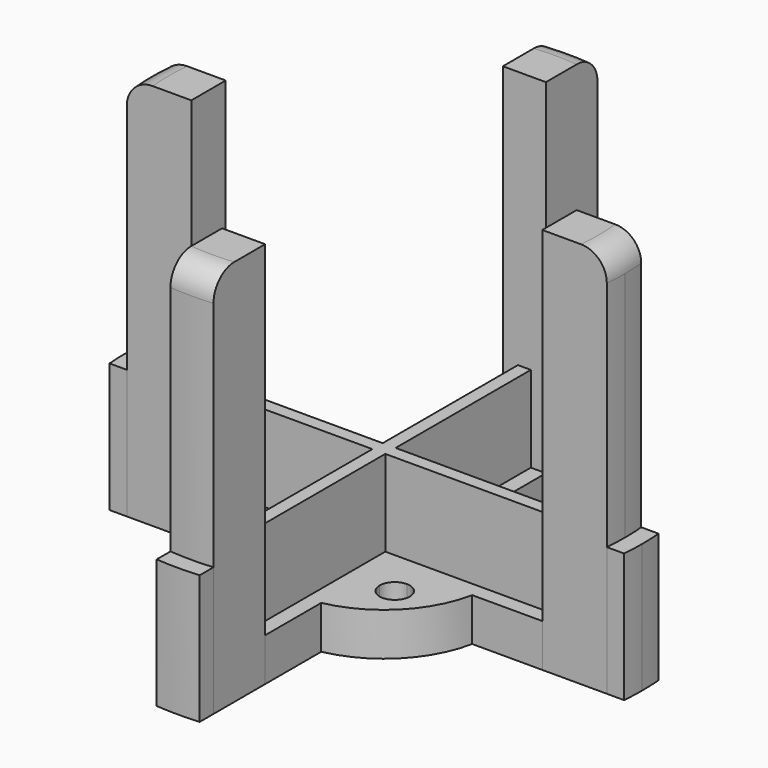
from build123d import *

# Parameters (mm, degrees)
F0_W          = 3.5
F0_H          = 7.5
F0_W_2        = 7.5
F0_H_2        = 3.5
F1_DEPTH      = 10
F0_W_3        = 3
F0_H_3        = 3
F2_DEPTH      = 30
F3_DEPTH      = 90
F4_T2_ANGLE   = 40.9393595263
F4_2_T2_ANGLE = 40.9393595263
F4_3_T2_ANGLE = 40.9393595263
F4_4_T2_ANGLE = 40.9393595263
F5_DEPTH      = 3


# Not quite as in the source:
# - a fillet or chamfer that OpenCascade refuses, or shapes differently, is made with other operations: its cross-section is extruded or revolved along the edge and cut away or added


with BuildPart() as f1:
    # F0 (on Top) → F1 (new body)
    with BuildSketch(Plane.XY):
        with BuildLine():
            Line((12.5, 5), (24.4948974278, 5))
            ThreePointArc((24.4948974278, 5), (17.6776695297, 17.6776695297), (5, 24.4948974278))
            Line((5, 24.4948974278), (5, 12.5))
            Line((5, 12.5), (9, 12.5))
            ThreePointArc((9, 12.5), (12.5, 16), (16, 12.5))
            ThreePointArc((16, 12.5), (14.9748737342, 10.0251262658), (12.5, 9))
            Line((12.5, 9), (12.5, 5))
        make_face()
        with BuildLine():
            Line((5, 12.5), (5, 24.4948974278))
            ThreePointArc((5, 24.4948974278), (3.2581304855, 24.7867824806), (1.5, 24.9549594269))
            Line((1.5, 24.9549594269), (1.5, 12.5))
            Line((1.5, 12.5), (5, 12.5))
        make_face()
        with Locations((3.25, 8.75)):
            Rectangle(F0_W, F0_H)
        with BuildLine():
            Line((5, 5), (12.5, 5))
            Line((12.5, 5), (12.5, 9))
            ThreePointArc((12.5, 9), (10.0251262658, 10.0251262658), (9, 12.5))
            Line((9, 12.5), (5, 12.5))
            Line((5, 12.5), (5, 5))
        make_face()
        with Locations((8.75, 3.25)):
            Rectangle(F0_W_2, F0_H_2)
        with Locations((3.25, 3.25)):
            Rectangle(F0_W, F0_H_2)
        with BuildLine():
            Line((5, 24.4948974278), (5, 40.7763390695))
            Line((5, 40.7763390695), (1.5, 40.7763390695))
            Line((1.5, 40.7763390695), (1.5, 24.9549594269))
            ThreePointArc((1.5, 24.9549594269), (3.2581304855, 24.7867824806), (5, 24.4948974278))
        make_face()
        with BuildLine():
            Line((40.7763390695, 1.5), (40.7763390695, 5))
            Line((40.7763390695, 5), (24.4948974278, 5))
            ThreePointArc((24.4948974278, 5), (24.7867824806, 3.2581304855), (24.9549594269, 1.5))
            Line((24.9549594269, 1.5), (40.7763390695, 1.5))
        make_face()
        with BuildLine():
            ThreePointArc((24.9549594269, 1.5), (24.7867824806, 3.2581304855), (24.4948974278, 5))
            Line((24.4948974278, 5), (12.5, 5))
            Line((12.5, 5), (12.5, 1.5))
            Line((12.5, 1.5), (24.9549594269, 1.5))
        make_face()
    extrude(amount=F1_DEPTH)


with BuildPart() as f1b:
    # F0 (on Top) → F1, piece 2 (new body)
    with BuildSketch(Plane.XY):
        with BuildLine():
            Line((-5, 12.5), (-5, 24.4948974278))
            ThreePointArc((-5, 24.4948974278), (-17.6776695297, 17.6776695297), (-24.4948974278, 5))
            Line((-24.4948974278, 5), (-12.5, 5))
            Line((-12.5, 5), (-12.5, 9))
            ThreePointArc((-12.5, 9), (-14.9748737342, 14.9748737342), (-9, 12.5))
            Line((-9, 12.5), (-5, 12.5))
        make_face()
        with BuildLine():
            Line((-5, 5), (-5, 12.5))
            Line((-5, 12.5), (-9, 12.5))
            ThreePointArc((-9, 12.5), (-10.0251262658, 10.0251262658), (-12.5, 9))
            Line((-12.5, 9), (-12.5, 5))
            Line((-12.5, 5), (-5, 5))
        make_face()
        with Locations((-8.75, 3.25)):
            Rectangle(F0_W_2, F0_H_2)
        with BuildLine():
            Line((-24.4948974278, 5), (-40.7763390695, 5))
            Line((-40.7763390695, 5), (-40.7763390695, 1.5))
            Line((-40.7763390695, 1.5), (-24.9549594269, 1.5))
            ThreePointArc((-24.9549594269, 1.5), (-24.7867824806, 3.2581304855), (-24.4948974278, 5))
        make_face()
        with BuildLine():
            Line((-1.5, 40.7763390695), (-5, 40.7763390695))
            Line((-5, 40.7763390695), (-5, 24.4948974278))
            ThreePointArc((-5, 24.4948974278), (-3.2581304855, 24.7867824806), (-1.5, 24.9549594269))
            Line((-1.5, 24.9549594269), (-1.5, 40.7763390695))
        make_face()
        with BuildLine():
            ThreePointArc((-1.5, 24.9549594269), (-3.2581304855, 24.7867824806), (-5, 24.4948974278))
            Line((-5, 24.4948974278), (-5, 12.5))
            Line((-5, 12.5), (-1.5, 12.5))
            Line((-1.5, 12.5), (-1.5, 24.9549594269))
        make_face()
        with Locations((-3.25, 8.75)):
            Rectangle(F0_W, F0_H)
        with Locations((-3.25, 3.25)):
            Rectangle(F0_W, F0_H_2)
        with BuildLine():
            Line((-12.5, 5), (-24.4948974278, 5))
            ThreePointArc((-24.4948974278, 5), (-24.7867824806, 3.2581304855), (-24.9549594269, 1.5))
            Line((-24.9549594269, 1.5), (-12.5, 1.5))
            Line((-12.5, 1.5), (-12.5, 5))
        make_face()
    extrude(amount=F1_DEPTH)


with BuildPart() as f1c:
    # F0 (on Top) → F1, piece 3 (new body)
    with BuildSketch(Plane.XY):
        with BuildLine():
            ThreePointArc((-24.9549594269, -1.5), (-24.7867824806, -3.2581304855), (-24.4948974278, -5))
            Line((-24.4948974278, -5), (-12.5, -5))
            Line((-12.5, -5), (-12.5, -1.5))
            Line((-12.5, -1.5), (-24.9549594269, -1.5))
        make_face()
        with BuildLine():
            ThreePointArc((-24.4948974278, -5), (-17.6776695297, -17.6776695297), (-5, -24.4948974278))
            Line((-5, -24.4948974278), (-5, -12.5))
            Line((-5, -12.5), (-9, -12.5))
            ThreePointArc((-9, -12.5), (-14.9748737342, -14.9748737342), (-12.5, -9))
            Line((-12.5, -9), (-12.5, -5))
            Line((-12.5, -5), (-24.4948974278, -5))
        make_face()
        with BuildLine():
            Line((-9, -12.5), (-5, -12.5))
            Line((-5, -12.5), (-5, -5))
            Line((-5, -5), (-12.5, -5))
            Line((-12.5, -5), (-12.5, -9))
            ThreePointArc((-12.5, -9), (-10.0251262658, -10.0251262658), (-9, -12.5))
        make_face()
        with BuildLine():
            Line((-5, -24.4948974278), (-5, -40.7763390695))
            Line((-5, -40.7763390695), (-1.5, -40.7763390695))
            Line((-1.5, -40.7763390695), (-1.5, -24.9549594269))
            ThreePointArc((-1.5, -24.9549594269), (-3.2581304855, -24.7867824806), (-5, -24.4948974278))
        make_face()
        with BuildLine():
            Line((-40.7763390695, -1.5), (-40.7763390695, -5))
            Line((-40.7763390695, -5), (-24.4948974278, -5))
            ThreePointArc((-24.4948974278, -5), (-24.7867824806, -3.2581304855), (-24.9549594269, -1.5))
            Line((-24.9549594269, -1.5), (-40.7763390695, -1.5))
        make_face()
        with Locations((-3.25, -8.75)):
            Rectangle(F0_W, F0_H)
        with BuildLine():
            Line((-5, -12.5), (-5, -24.4948974278))
            ThreePointArc((-5, -24.4948974278), (-3.2581304855, -24.7867824806), (-1.5, -24.9549594269))
            Line((-1.5, -24.9549594269), (-1.5, -12.5))
            Line((-1.5, -12.5), (-5, -12.5))
        make_face()
        with Locations((-8.75, -3.25)):
            Rectangle(F0_W_2, F0_H_2)
        with Locations((-3.25, -3.25)):
            Rectangle(F0_W, F0_H_2)
    extrude(amount=F1_DEPTH)


with BuildPart() as f1d:
    # F0 (on Top) → F1, piece 4 (new body)
    with BuildSketch(Plane.XY):
        with Locations((3.25, -8.75)):
            Rectangle(F0_W, F0_H)
        with BuildLine():
            Line((12.5, -9), (12.5, -5))
            Line((12.5, -5), (5, -5))
            Line((5, -5), (5, -12.5))
            Line((5, -12.5), (9, -12.5))
            ThreePointArc((9, -12.5), (10.0251262658, -10.0251262658), (12.5, -9))
        make_face()
        with BuildLine():
            ThreePointArc((5, -24.4948974278), (17.6776695297, -17.6776695297), (24.4948974278, -5))
            Line((24.4948974278, -5), (12.5, -5))
            Line((12.5, -5), (12.5, -9))
            ThreePointArc((12.5, -9), (14.9748737342, -10.0251262658), (16, -12.5))
            ThreePointArc((16, -12.5), (12.5, -16), (9, -12.5))
            Line((9, -12.5), (5, -12.5))
            Line((5, -12.5), (5, -24.4948974278))
        make_face()
        with BuildLine():
            Line((12.5, -5), (24.4948974278, -5))
            ThreePointArc((24.4948974278, -5), (24.7867824806, -3.2581304855), (24.9549594269, -1.5))
            Line((24.9549594269, -1.5), (12.5, -1.5))
            Line((12.5, -1.5), (12.5, -5))
        make_face()
        with BuildLine():
            ThreePointArc((1.5, -24.9549594269), (3.2581304855, -24.7867824806), (5, -24.4948974278))
            Line((5, -24.4948974278), (5, -12.5))
            Line((5, -12.5), (1.5, -12.5))
            Line((1.5, -12.5), (1.5, -24.9549594269))
        make_face()
        with BuildLine():
            Line((1.5, -40.7763390695), (5, -40.7763390695))
            Line((5, -40.7763390695), (5, -24.4948974278))
            ThreePointArc((5, -24.4948974278), (3.2581304855, -24.7867824806), (1.5, -24.9549594269))
            Line((1.5, -24.9549594269), (1.5, -40.7763390695))
        make_face()
        with BuildLine():
            Line((24.4948974278, -5), (40.7763390695, -5))
            Line((40.7763390695, -5), (40.7763390695, -1.5))
            Line((40.7763390695, -1.5), (24.9549594269, -1.5))
            ThreePointArc((24.9549594269, -1.5), (24.7867824806, -3.2581304855), (24.4948974278, -5))
        make_face()
        with Locations((3.25, -3.25)):
            Rectangle(F0_W, F0_H_2)
        with Locations((8.75, -3.25)):
            Rectangle(F0_W_2, F0_H_2)
    extrude(amount=F1_DEPTH)


with BuildPart() as f2:
    # F0 (on Top) → F2 (new body)
    with BuildSketch(Plane.XY):
        with BuildLine():
            Line((1.5, 24.9549594269), (1.5, 40.7763390695))
            Line((1.5, 40.7763390695), (-1.5, 40.7763390695))
            Line((-1.5, 40.7763390695), (-1.5, 24.9549594269))
            ThreePointArc((-1.5, 24.9549594269), (0, 25), (1.5, 24.9549594269))
        make_face()
        with BuildLine():
            Line((1.5, 12.5), (1.5, 24.9549594269))
            ThreePointArc((1.5, 24.9549594269), (0, 25), (-1.5, 24.9549594269))
            Line((-1.5, 24.9549594269), (-1.5, 12.5))
            Line((-1.5, 12.5), (1.5, 12.5))
        make_face()
        with Locations((0, 8.75)):
            Rectangle(F0_W_3, F0_H)
        with Locations((0, 3.25)):
            Rectangle(F0_W_3, F0_H_2)
        Rectangle(F0_W_3, F0_H_3)
        with Locations((0, -3.25)):
            Rectangle(F0_W_3, F0_H_2)
        with Locations((0, -8.75)):
            Rectangle(F0_W_3, F0_H)
        with BuildLine():
            ThreePointArc((-1.5, -24.9549594269), (0, -25), (1.5, -24.9549594269))
            Line((1.5, -24.9549594269), (1.5, -12.5))
            Line((1.5, -12.5), (-1.5, -12.5))
            Line((-1.5, -12.5), (-1.5, -24.9549594269))
        make_face()
        with BuildLine():
            Line((-1.5, -40.7763390695), (1.5, -40.7763390695))
            Line((1.5, -40.7763390695), (1.5, -24.9549594269))
            ThreePointArc((1.5, -24.9549594269), (0, -25), (-1.5, -24.9549594269))
            Line((-1.5, -24.9549594269), (-1.5, -40.7763390695))
        make_face()
        with Locations((8.75, 0)):
            Rectangle(F0_W_2, F0_H_3)
        with BuildLine():
            ThreePointArc((25, 0), (24.9887373198, 0.7503380327), (24.9549594269, 1.5))
            Line((24.9549594269, 1.5), (12.5, 1.5))
            Line((12.5, 1.5), (12.5, -1.5))
            Line((12.5, -1.5), (24.9549594269, -1.5))
            ThreePointArc((24.9549594269, -1.5), (24.9887373198, -0.7503380327), (25, 0))
        make_face()
        with BuildLine():
            Line((40.7763390695, -1.5), (40.7763390695, 1.5))
            Line((40.7763390695, 1.5), (24.9549594269, 1.5))
            ThreePointArc((24.9549594269, 1.5), (24.9887373198, 0.7503380327), (25, 0))
            ThreePointArc((25, 0), (24.9887373198, -0.7503380327), (24.9549594269, -1.5))
            Line((24.9549594269, -1.5), (40.7763390695, -1.5))
        make_face()
        with Locations((-3.25, 0)):
            Rectangle(F0_W, F0_H_3)
        with Locations((-8.75, 0)):
            Rectangle(F0_W_2, F0_H_3)
        with BuildLine():
            Line((-12.5, 1.5), (-24.9549594269, 1.5))
            ThreePointArc((-24.9549594269, 1.5), (-25, 0), (-24.9549594269, -1.5))
            Line((-24.9549594269, -1.5), (-12.5, -1.5))
            Line((-12.5, -1.5), (-12.5, 1.5))
        make_face()
        with BuildLine():
            Line((-24.9549594269, 1.5), (-40.7763390695, 1.5))
            Line((-40.7763390695, 1.5), (-40.7763390695, -1.5))
            Line((-40.7763390695, -1.5), (-24.9549594269, -1.5))
            ThreePointArc((-24.9549594269, -1.5), (-25, 0), (-24.9549594269, 1.5))
        make_face()
        with Locations((3.25, 0)):
            Rectangle(F0_W, F0_H_3)
    extrude(amount=F2_DEPTH)


with BuildPart() as f2b:
    # F0 (on Top) → F2, piece 2 (new body)
    with BuildSketch(Plane.XY):
        with BuildLine():
            Line((-55.7763390695, 5), (-59.7913037155, 5))
            ThreePointArc((-59.7913037155, 5), (-60, 0), (-59.7913037155, -5))
            Line((-59.7913037155, -5), (-55.7763390695, -5))
            ThreePointArc((-55.7763390695, -5), (-56, 0), (-55.7763390695, 5))
        make_face()
    extrude(amount=F2_DEPTH)


with BuildPart() as f2c:
    # F0 (on Top) → F2, piece 3 (new body)
    with BuildSketch(Plane.XY):
        with BuildLine():
            ThreePointArc((59.7913037155, -5), (59.9478032247, -2.5021767593), (60, 0))
            ThreePointArc((60, 0), (59.9478032247, 2.5021767593), (59.7913037155, 5))
            Line((59.7913037155, 5), (55.7763390695, 5))
            ThreePointArc((55.7763390695, 5), (55.9440568242, 2.5024999606), (56, 0))
            ThreePointArc((56, 0), (55.9440568242, -2.5024999606), (55.7763390695, -5))
            Line((55.7763390695, -5), (59.7913037155, -5))
        make_face()
    extrude(amount=F2_DEPTH)


with BuildPart() as f2d:
    # F0 (on Top) → F2, piece 4 (new body)
    with BuildSketch(Plane.XY):
        with BuildLine():
            Line((5, 55.7763390695), (5, 59.7913037155))
            ThreePointArc((5, 59.7913037155), (0, 60), (-5, 59.7913037155))
            Line((-5, 59.7913037155), (-5, 55.7763390695))
            ThreePointArc((-5, 55.7763390695), (0, 56), (5, 55.7763390695))
        make_face()
    extrude(amount=F2_DEPTH)


with BuildPart() as f2e:
    # F0 (on Top) → F2, piece 5 (new body)
    with BuildSketch(Plane.XY):
        with BuildLine():
            ThreePointArc((-5, -59.7913037155), (0, -60), (5, -59.7913037155))
            Line((5, -59.7913037155), (5, -55.7763390695))
            ThreePointArc((5, -55.7763390695), (0, -56), (-5, -55.7763390695))
            Line((-5, -55.7763390695), (-5, -59.7913037155))
        make_face()
    extrude(amount=F2_DEPTH)


with BuildPart() as f3:
    # F0 (on Top) → F3 (new body)
    with BuildSketch(Plane.XY):
        Polygon((5, 40.7763390695), (5, 55.7763390695), (-5, 55.7763390695), (-5, 40.7763390695), (-1.5, 40.7763390695), (1.5, 40.7763390695), align=None)
        with BuildLine():
            Line((-5, 55.7763390695), (5, 55.7763390695))
            ThreePointArc((5, 55.7763390695), (0, 56), (-5, 55.7763390695))
        make_face()
    extrude(amount=F3_DEPTH)

    # F4: fillet of radius 6 on 1 edges, made by hand

    # F4_s1 → F4_t2 (revolve, cut)
    with BuildSketch(Plane(origin=(0, 0, 0), x_dir=(0, 0, 1), z_dir=(0.9368573836, -0.3497116566, 0))):
        with BuildLine():
            ThreePointArc((84, -56), (88.2426406871, -54.2426406871), (90, -50))
            Line((90, -50), (90, -56))
            Line((90, -56), (84, -56))
        make_face()
    revolve(axis=Axis((0, 0, 90), (0, 0, 1)), revolution_arc=F4_T2_ANGLE, mode=Mode.SUBTRACT)


with BuildPart() as f3b:
    # F0 (on Top) → F3, piece 2 (new body)
    with BuildSketch(Plane.XY):
        Polygon((-40.7763390695, 5), (-55.7763390695, 5), (-55.7763390695, -5), (-40.7763390695, -5), (-40.7763390695, -1.5), (-40.7763390695, 1.5), align=None)
        with BuildLine():
            Line((-55.7763390695, -5), (-55.7763390695, 5))
            ThreePointArc((-55.7763390695, 5), (-56, 0), (-55.7763390695, -5))
        make_face()
    extrude(amount=F3_DEPTH)

    # F4#2: fillet of radius 6 on 1 edges, made by hand

    # F4_2_s1 → F4_2_t2 (revolve, cut)
    with BuildSketch(Plane(origin=(0, 0, 0), x_dir=(0, 0, 1), z_dir=(0.3497116566, 0.9368573836, 0))):
        with BuildLine():
            ThreePointArc((84, -56), (88.2426406871, -54.2426406871), (90, -50))
            Line((90, -50), (90, -56))
            Line((90, -56), (84, -56))
        make_face()
    revolve(axis=Axis((0, 0, 90), (0, 0, 1)), revolution_arc=F4_2_T2_ANGLE, mode=Mode.SUBTRACT)


with BuildPart() as f3c:
    # F0 (on Top) → F3, piece 3 (new body)
    with BuildSketch(Plane.XY):
        Polygon((-5, -55.7763390695), (5, -55.7763390695), (5, -40.7763390695), (1.5, -40.7763390695), (-1.5, -40.7763390695), (-5, -40.7763390695), align=None)
        with BuildLine():
            ThreePointArc((-5, -55.7763390695), (0, -56), (5, -55.7763390695))
            Line((5, -55.7763390695), (-5, -55.7763390695))
        make_face()
    extrude(amount=F3_DEPTH)

    # F4#3: fillet of radius 6 on 1 edges, made by hand

    # F4_3_s1 → F4_3_t2 (revolve, cut)
    with BuildSketch(Plane(origin=(0, 0, 0), x_dir=(0, 0, 1), z_dir=(-0.9368573836, 0.3497116566, 0))):
        with BuildLine():
            ThreePointArc((84, -56), (88.2426406871, -54.2426406871), (90, -50))
            Line((90, -50), (90, -56))
            Line((90, -56), (84, -56))
        make_face()
    revolve(axis=Axis((0, 0, 90), (0, 0, 1)), revolution_arc=F4_3_T2_ANGLE, mode=Mode.SUBTRACT)


with BuildPart() as f3d:
    # F0 (on Top) → F3, piece 4 (new body)
    with BuildSketch(Plane.XY):
        Polygon((55.7763390695, -5), (55.7763390695, 5), (40.7763390695, 5), (40.7763390695, 1.5), (40.7763390695, -1.5), (40.7763390695, -5), align=None)
        with BuildLine():
            ThreePointArc((56, 0), (55.9440568242, 2.5024999606), (55.7763390695, 5))
            Line((55.7763390695, 5), (55.7763390695, -5))
            ThreePointArc((55.7763390695, -5), (55.9440568242, -2.5024999606), (56, 0))
        make_face()
    extrude(amount=F3_DEPTH)

    # F4#4: fillet of radius 6 on 1 edges, made by hand

    # F4_4_s1 → F4_4_t2 (revolve, cut)
    with BuildSketch(Plane(origin=(0, 0, 0), x_dir=(0, 0, 1), z_dir=(-0.3497116566, -0.9368573836, 0))):
        with BuildLine():
            ThreePointArc((84, -56), (88.2426406871, -54.2426406871), (90, -50))
            Line((90, -50), (90, -56))
            Line((90, -56), (84, -56))
        make_face()
    revolve(axis=Axis((0, 0, 90), (0, 0, 1)), revolution_arc=F4_4_T2_ANGLE, mode=Mode.SUBTRACT)


with BuildPart() as f5:
    # F0 (on Top) → F5 (new body)
    with BuildSketch(Plane.XY):
        with BuildLine():
            Line((-10.75, 12.5), (-9, 12.5))
            ThreePointArc((-9, 12.5), (-14.9748737342, 14.9748737342), (-12.5, 9))
            Line((-12.5, 9), (-12.5, 10.75))
            ThreePointArc((-12.5, 10.75), (-13.7374368671, 13.7374368671), (-10.75, 12.5))
        make_face()
        with BuildLine():
            ThreePointArc((-12.5, 9), (-10.0251262658, 10.0251262658), (-9, 12.5))
            Line((-9, 12.5), (-10.75, 12.5))
            ThreePointArc((-10.75, 12.5), (-11.2625631329, 11.2625631329), (-12.5, 10.75))
            Line((-12.5, 10.75), (-12.5, 9))
        make_face()
    extrude(amount=F5_DEPTH)


with BuildPart() as f5b:
    # F0 (on Top) → F5, piece 2 (new body)
    with BuildSketch(Plane.XY):
        with BuildLine():
            Line((12.5, 10.75), (12.5, 9))
            ThreePointArc((12.5, 9), (14.9748737342, 10.0251262658), (16, 12.5))
            ThreePointArc((16, 12.5), (12.5, 16), (9, 12.5))
            Line((9, 12.5), (10.75, 12.5))
            ThreePointArc((10.75, 12.5), (12.5, 14.25), (14.25, 12.5))
            ThreePointArc((14.25, 12.5), (13.7374368671, 11.2625631329), (12.5, 10.75))
        make_face()
        with BuildLine():
            ThreePointArc((9, 12.5), (10.0251262658, 10.0251262658), (12.5, 9))
            Line((12.5, 9), (12.5, 10.75))
            ThreePointArc((12.5, 10.75), (11.2625631329, 11.2625631329), (10.75, 12.5))
            Line((10.75, 12.5), (9, 12.5))
        make_face()
    extrude(amount=F5_DEPTH)


with BuildPart() as f5c:
    # F0 (on Top) → F5, piece 3 (new body)
    with BuildSketch(Plane.XY):
        with BuildLine():
            ThreePointArc((-12.5, -9), (-14.9748737342, -14.9748737342), (-9, -12.5))
            Line((-9, -12.5), (-10.75, -12.5))
            ThreePointArc((-10.75, -12.5), (-13.7374368671, -13.7374368671), (-12.5, -10.75))
            Line((-12.5, -10.75), (-12.5, -9))
        make_face()
        with BuildLine():
            Line((-10.75, -12.5), (-9, -12.5))
            ThreePointArc((-9, -12.5), (-10.0251262658, -10.0251262658), (-12.5, -9))
            Line((-12.5, -9), (-12.5, -10.75))
            ThreePointArc((-12.5, -10.75), (-11.2625631329, -11.2625631329), (-10.75, -12.5))
        make_face()
    extrude(amount=F5_DEPTH)


with BuildPart() as f5d:
    # F0 (on Top) → F5, piece 4 (new body)
    with BuildSketch(Plane.XY):
        with BuildLine():
            ThreePointArc((16, -12.5), (14.9748737342, -10.0251262658), (12.5, -9))
            Line((12.5, -9), (12.5, -10.75))
            ThreePointArc((12.5, -10.75), (13.7374368671, -11.2625631329), (14.25, -12.5))
            ThreePointArc((14.25, -12.5), (12.5, -14.25), (10.75, -12.5))
            Line((10.75, -12.5), (9, -12.5))
            ThreePointArc((9, -12.5), (12.5, -16), (16, -12.5))
        make_face()
        with BuildLine():
            Line((12.5, -10.75), (12.5, -9))
            ThreePointArc((12.5, -9), (10.0251262658, -10.0251262658), (9, -12.5))
            Line((9, -12.5), (10.75, -12.5))
            ThreePointArc((10.75, -12.5), (11.2625631329, -11.2625631329), (12.5, -10.75))
        make_face()
    extrude(amount=F5_DEPTH)


solid = Compound([f1.part, f1b.part, f1c.part, f1d.part, f2.part, f2b.part, f2c.part, f2d.part, f2e.part, f3.part, f3b.part, f3c.part, f3d.part, f5.part, f5b.part, f5c.part, f5d.part])
